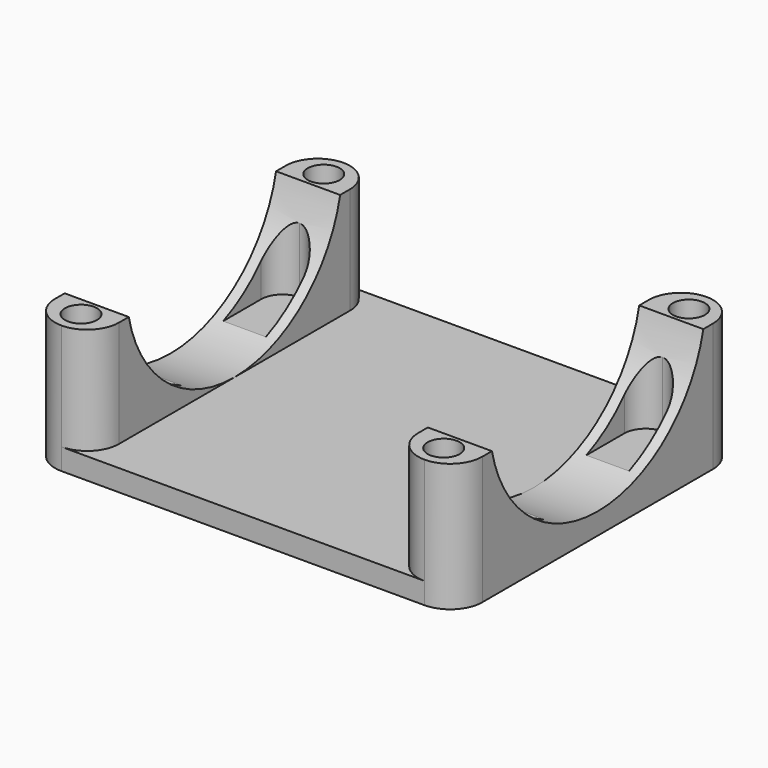
from build123d import *

# Parameters (mm, degrees)
F0_W      = 40
F0_H      = 33
F1_DEPTH  = 12
F2_R      = 12.65
F3_DEPTH  = 69
F4_W      = 28
F4_H      = 48.7952879344
F5_DEPTH  = 10
F7_DEPTH  = 9
F8_R      = 2.99999
F9_R      = 1.5
F10_DEPTH = 20


# Not quite as in the source:
# - a fillet or chamfer is up to 0.001 mm smaller than in the source, because OpenCascade refuses the exact size


with BuildPart() as f1:
    # F0 (on Top) → F1 (new body)
    with BuildSketch(Plane.XY):
        with Locations((-8.7267248217, -1.6879990697)):
            Rectangle(F0_W, F0_H)
    extrude(amount=F1_DEPTH)

    # F2 (on face) → F3 (cut)
    with BuildSketch(Plane.YZ.offset(11.2732751783)):
        with Locations((-1.6879990697, 14.65)):
            Circle(F2_R)
    extrude(amount=-F3_DEPTH, mode=Mode.SUBTRACT)

    # F4 (on face) → F5 (cut)
    with BuildSketch(Plane.XY.offset(12)):
        with Locations((-8.7267248217, 5.2832299843)):
            Rectangle(F4_W, F4_H)
    extrude(amount=-F5_DEPTH, mode=Mode.SUBTRACT)

    # F6 (on face) → F7 (cut)
    with BuildSketch(Plane.XY.offset(12)):
        with BuildLine():
            ThreePointArc((-25.7267248217, 9.6813178072), (-27.140938384, 9.0955313695), (-27.7267248217, 7.6813178072))
            Line((-27.7267248217, 7.6813178072), (-27.7267248217, -11.0573159465))
            ThreePointArc((-27.7267248217, -11.0573159465), (-27.140938384, -12.4715295089), (-25.7267248217, -13.0573159465))
            ThreePointArc((-25.7267248217, -13.0573159465), (-24.3125112593, -12.4715295089), (-23.7267248217, -11.0573159465))
            Line((-23.7267248217, -11.0573159465), (-23.7267248217, 7.6813178072))
            ThreePointArc((-23.7267248217, 7.6813178072), (-24.3125112593, 9.0955313695), (-25.7267248217, 9.6813178072))
        make_face()
        with BuildLine():
            ThreePointArc((8.2732751783, 9.6813178072), (6.859061616, 9.0955313695), (6.2732751783, 7.6813178072))
            Line((6.2732751783, 7.6813178072), (6.2732751783, -11.0573159465))
            ThreePointArc((6.2732751783, -11.0573159465), (6.859061616, -12.4715295089), (8.2732751783, -13.0573159465))
            ThreePointArc((8.2732751783, -13.0573159465), (9.6874887407, -12.4715295089), (10.2732751783, -11.0573159465))
            Line((10.2732751783, -11.0573159465), (10.2732751783, 7.6813178072))
            ThreePointArc((10.2732751783, 7.6813178072), (9.6874887407, 9.0955313695), (8.2732751783, 9.6813178072))
        make_face()
    extrude(amount=-F7_DEPTH, mode=Mode.SUBTRACT)

    # F8 (radius 3 in the source; OpenCascade refuses exactly that, so slightly less here)
    f8_edges = [f1.edges().sort_by_distance(p)[0] for p in [
        (5.273275, 14.812001, 7),
        (11.273275, 14.812001, 6),
        (-22.726725, 14.812001, 7),
        (-28.726725, 14.812001, 6),
        (-28.726725, -18.187999, 6),
        (-22.726725, -18.187999, 7),
        (5.273275, -18.187999, 7),
        (11.273275, -18.187999, 6),
    ]]
    fillet(f8_edges, radius=F8_R)

    # F9 (on face) → F10 (cut)
    with BuildSketch(Plane.XY.offset(12)):
        with Locations((-25.7267248217, 12.5120009303)):
            Circle(F9_R)
        with Locations((8.4634907544, 12.5120009303)):
            Circle(F9_R)
        with Locations((8.2223585095, -15.8879990697)):
            Circle(F9_R)
        with Locations((-25.7357346928, -15.8880167171)):
            Circle(F9_R)
    extrude(amount=-F10_DEPTH, mode=Mode.SUBTRACT)


solid = f1.part
